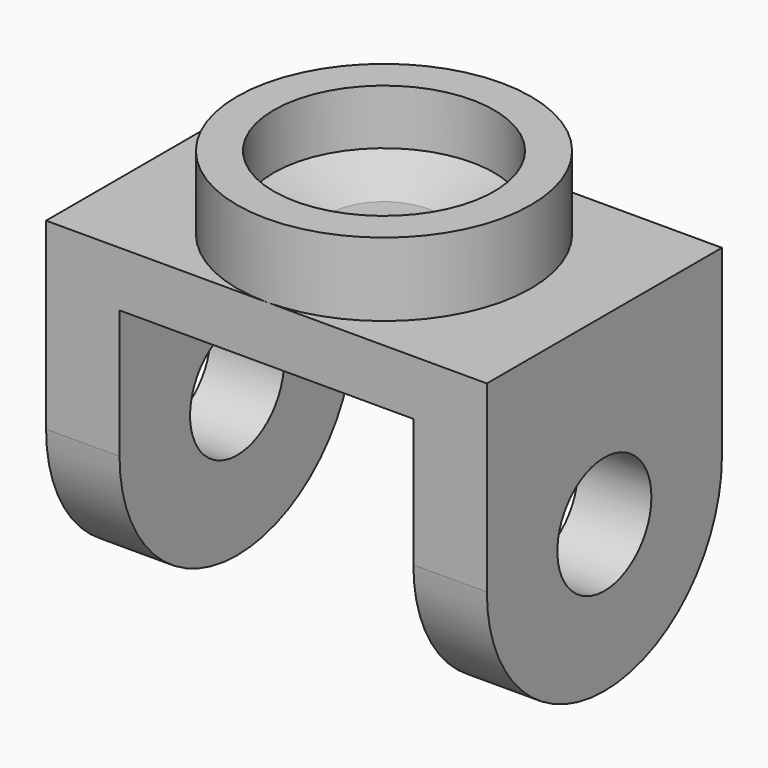
from build123d import *

# Parameters (mm, degrees)
F0_R     = 30
F0_R_2   = 15
F1_DEPTH = 90
F2_R     = 16
F3_DEPTH = 250
F4_DEPTH = 250
F5_DEPTH = 250
F6_W     = 80
F6_H     = 40
F6_H_2   = 35
F7_DEPTH = 250
F8_DEPTH = 25


# Not quite as in the source:
# - a feature names something its author has since deleted; it is built from what else it names


with BuildPart() as f1:
    # F0 (on Top) → F1 (new body)
    with BuildSketch(Plane.XY):
        with BuildLine():
            Line((0, -40), (60, -40))
            Line((60, -40), (60, 40))
            Line((60, 40), (0, 40))
            ThreePointArc((0, 40), (28.2842712475, 28.2842712475), (40, 0))
            ThreePointArc((40, 0), (28.2842712475, -28.2842712475), (0, -40))
        make_face()
        with BuildLine():
            Line((-60, -40), (0, -40))
            ThreePointArc((0, -40), (-40, 0), (0, 40))
            Line((0, 40), (-60, 40))
            Line((-60, 40), (-60, -40))
        make_face()
        with BuildLine():
            ThreePointArc((0, 40), (-40, 0), (0, -40))
            ThreePointArc((0, -40), (28.2842712475, -28.2842712475), (40, 0))
            ThreePointArc((40, 0), (28.2842712475, 28.2842712475), (0, 40))
        make_face()
        Circle(F0_R, mode=Mode.SUBTRACT)
        Circle(F0_R)
        Circle(F0_R_2, mode=Mode.SUBTRACT)
        Circle(F0_R_2)
    extrude(amount=-F1_DEPTH)

    # F2 (on face) → F3 (cut)
    with BuildSketch(Plane.YZ.offset(60)):
        with BuildLine():
            ThreePointArc((0, -90), (-28.2842712475, -78.2842712475), (-40, -50))
            Line((-40, -50), (-40, -90))
            Line((-40, -90), (0, -90))
        make_face()
        with BuildLine():
            Line((40, -90), (40, -50))
            ThreePointArc((40, -50), (28.2842712475, -78.2842712475), (0, -90))
            Line((0, -90), (40, -90))
        make_face()
        with Locations((0, -50)):
            Circle(F2_R)
    extrude(amount=-F3_DEPTH, mode=Mode.SUBTRACT)

    # F2 (on face) → F4 (cut)
    with BuildSketch(Plane.YZ.offset(60)):
        with Locations((0, -50)):
            Circle(F2_R)
    extrude(amount=-F4_DEPTH, mode=Mode.SUBTRACT)

    # F2 (on face) → F5 (cut)
    with BuildSketch(Plane.YZ.offset(60)):
        with Locations((0, -50)):
            Circle(F2_R)
    extrude(amount=-F5_DEPTH, mode=Mode.SUBTRACT)

    # F6 (on face) → F7 (cut)
    with BuildSketch(Plane.XZ.offset(40)):
        with Locations((0, -70)):
            Rectangle(F6_W, F6_H)
        with Locations((0, -32.5)):
            Rectangle(F6_W, F6_H_2)
    extrude(amount=-F7_DEPTH, mode=Mode.SUBTRACT)

    # F2 (on face) → F8 (cut)
    with BuildSketch(Plane.YZ.offset(60)):
        with BuildLine():
            ThreePointArc((0, -90), (-28.2842712475, -78.2842712475), (-40, -50))
            Line((-40, -50), (-40, -90))
            Line((-40, -90), (0, -90))
        make_face()
    extrude(amount=-F8_DEPTH, mode=Mode.SUBTRACT)


with BuildPart() as f10:
    # F9 (on Front) → F10 (revolve)
    with BuildSketch(Plane.XZ):
        Polygon((-40, 20), (-40, 0), (-15, 0), (-30, 5), (-30, 20), align=None)
    revolve(axis=Axis((0, 0, 21.7640828341), (0, 0, 1)))


solid = Compound([f1.part, f10.part])
